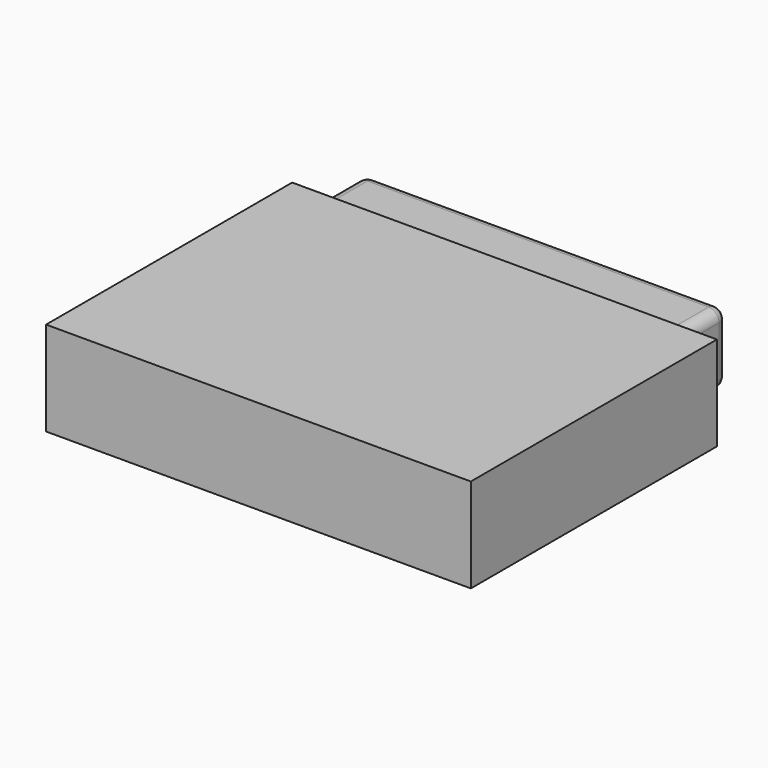
from build123d import *

# Parameters (mm, degrees)
F0_W         = 203
F0_H         = 147
F1_DEPTH     = 45
F2_R         = 7
F3_DEPTH     = 3
F4_R         = 9
F5_DEPTH     = 10
F6_W         = 173
F6_H         = 34
F7_DEPTH     = 25
F8_T1_DEPTH  = 163
F8_T3_DEPTH  = 24
F8_T5_DEPTH  = 20
F8_S9_W      = 5
F8_S9_H      = 5
F8_T10_DEPTH = 5
F8_S15_W     = 5
F8_S15_H     = 5
F8_T16_DEPTH = 5
F8_S21_W     = 5
F8_S21_H     = 5
F8_T22_DEPTH = 5
F8_S27_W     = 5
F8_S27_H     = 5
F8_T28_DEPTH = 5
F8_T34_DEPTH = 22.5
F8_S36_R     = 9
F8_T37_DEPTH = 13
F8_T42_DEPTH = 10
F8_S43_R     = 9
F8_T44_DEPTH = 8
F8_T48_DEPTH = 10
F8_S49_R     = 9
F8_T50_DEPTH = 8
F9_W         = 18
F9_H         = 30
F10_DEPTH    = 10


# Not quite as in the source:
# - a fillet or chamfer that OpenCascade refuses, or shapes differently, is made with other operations: its cross-section is extruded or revolved along the edge and cut away or added


with BuildPart() as f1:
    # F0 (on Top) → F1 (new body)
    with BuildSketch(Plane.XY):
        with Locations((0, 73.5)):
            Rectangle(F0_W, F0_H)
    extrude(amount=F1_DEPTH)

    # F2 (on face) → F3 (join)
    with BuildSketch(Plane(origin=(0, 0, 0), x_dir=(1, 0, 0), z_dir=(0, 0, -1))):
        with Locations((-88.5, -14)):
            Circle(F2_R)
        with Locations((-88.5, -117)):
            Circle(F2_R)
        with Locations((88.5, -14)):
            Circle(F2_R)
        with Locations((88.5, -117)):
            Circle(F2_R)
    extrude(amount=F3_DEPTH)

    # F4 (on face) → F5 (join)
    with BuildSketch(Plane(origin=(0, 147, 0), x_dir=(-1, 0, 0), z_dir=(0, 1, 0))):
        with Locations((91, 8)):
            Circle(F4_R)
    extrude(amount=F5_DEPTH)

    # F6 (on face) → F7 (join)
    with BuildSketch(Plane(origin=(0, 147, 0), x_dir=(-1, 0, 0), z_dir=(0, 1, 0))):
        with Locations((0, 27)):
            Rectangle(F6_W, F6_H)
    extrude(amount=F7_DEPTH)

    # F8: fillet of radius 5 on 8 edges, made by hand

    # F8_s2 → F8_t1 (cut)
    with BuildSketch(Plane.YZ.offset(-81.5)):
        with BuildLine():
            ThreePointArc((172, 39), (170.5355339059, 42.5355339059), (167, 44))
            Line((167, 44), (172, 44))
            Line((172, 44), (172, 39))
        make_face()
        with BuildLine():
            ThreePointArc((167, 10), (170.5355339059, 11.4644660941), (172, 15))
            Line((172, 15), (172, 10))
            Line((172, 10), (167, 10))
        make_face()
    extrude(amount=F8_T1_DEPTH, mode=Mode.SUBTRACT)

    # F8_s4 → F8_t3 (cut)
    with BuildSketch(Plane.XY.offset(15)):
        with BuildLine():
            ThreePointArc((81.5, 172), (85.0355339059, 170.5355339059), (86.5, 167))
            Line((86.5, 167), (86.5, 172))
            Line((86.5, 172), (81.5, 172))
        make_face()
        with BuildLine():
            ThreePointArc((-81.5, 172), (-85.0355339059, 170.5355339059), (-86.5, 167))
            Line((-86.5, 167), (-86.5, 172))
            Line((-86.5, 172), (-81.5, 172))
        make_face()
    extrude(amount=F8_T3_DEPTH, mode=Mode.SUBTRACT)

    # F8_s6 → F8_t5 (cut)
    with BuildSketch(Plane.XZ.offset(-167)):
        with BuildLine():
            ThreePointArc((86.5, 39), (85.0355339059, 42.5355339059), (81.5, 44))
            Line((81.5, 44), (86.5, 44))
            Line((86.5, 44), (86.5, 39))
        make_face()
        with BuildLine():
            ThreePointArc((81.5, 10), (85.0355339059, 11.4644660941), (86.5, 15))
            Line((86.5, 15), (86.5, 10))
            Line((86.5, 10), (81.5, 10))
        make_face()
        with BuildLine():
            ThreePointArc((-81.5, 44), (-85.0355339059, 42.5355339059), (-86.5, 39))
            Line((-86.5, 39), (-86.5, 44))
            Line((-86.5, 44), (-81.5, 44))
        make_face()
    extrude(amount=F8_T5_DEPTH, mode=Mode.SUBTRACT)


with BuildPart() as f8_tool8:
    # F8_s9 → F8_t10 (new body)
    with BuildSketch(Plane.XZ.offset(-167)):
        with Locations((-84, 41.5)):
            Rectangle(F8_S9_W, F8_S9_H)
    extrude(amount=-F8_T10_DEPTH)

    # F8_s11 → F8_t12 (revolve, cut)
    with BuildSketch(Plane(origin=(-81.5, 167, 39), x_dir=(0.7071067812, 0, -0.7071067812), z_dir=(0.7071067812, 0, 0.7071067812))):
        with BuildLine():
            ThreePointArc((0, -5), (5, 0), (0, 5))
            Line((0, 5), (0, -5))
        make_face()
    revolve(axis=Axis((-81.5, 167, 39), (0, 1, 0)), mode=Mode.SUBTRACT)


with BuildPart() as f1_1:
    add(f1.part)

    # F8_t7: cut F8_tool8
    add(f8_tool8.part, mode=Mode.SUBTRACT)


with BuildPart() as f8_tool14:
    # F8_s15 → F8_t16 (new body)
    with BuildSketch(Plane.XZ.offset(-167)):
        with Locations((84, 41.5)):
            Rectangle(F8_S15_W, F8_S15_H)
    extrude(amount=-F8_T16_DEPTH)

    # F8_s17 → F8_t18 (revolve, cut)
    with BuildSketch(Plane(origin=(81.5, 167, 39), x_dir=(-0.7071067812, 0, -0.7071067812), z_dir=(0.7071067812, 0, -0.7071067812))):
        with BuildLine():
            ThreePointArc((0, -5), (5, 0), (0, 5))
            Line((0, 5), (0, -5))
        make_face()
    revolve(axis=Axis((81.5, 167, 39), (0, 1, 0)), mode=Mode.SUBTRACT)


with BuildPart() as f1_2:
    add(f1_1.part)

    # F8_t13: cut F8_tool14
    add(f8_tool14.part, mode=Mode.SUBTRACT)


with BuildPart() as f8_tool20:
    # F8_s21 → F8_t22 (new body)
    with BuildSketch(Plane.XY.offset(15)):
        with Locations((84, 169.5)):
            Rectangle(F8_S21_W, F8_S21_H)
    extrude(amount=-F8_T22_DEPTH)

    # F8_s23 → F8_t24 (revolve, cut)
    with BuildSketch(Plane(origin=(81.5, 167, 15), x_dir=(-0.7071067812, -0.7071067812, 0), z_dir=(0.7071067812, -0.7071067812, 0))):
        with BuildLine():
            ThreePointArc((0, -5), (5, 0), (0, 5))
            Line((0, 5), (0, -5))
        make_face()
    revolve(axis=Axis((81.5, 167, 15), (0, 0, -1)), mode=Mode.SUBTRACT)


with BuildPart() as f1_3:
    add(f1_2.part)

    # F8_t19: cut F8_tool20
    add(f8_tool20.part, mode=Mode.SUBTRACT)


with BuildPart() as f8_tool26:
    # F8_s27 → F8_t28 (new body)
    with BuildSketch(Plane.XY.offset(15)):
        with Locations((-84, 169.5)):
            Rectangle(F8_S27_W, F8_S27_H)
    extrude(amount=-F8_T28_DEPTH)

    # F8_s29 → F8_t30 (revolve, cut)
    with BuildSketch(Plane(origin=(-81.5, 167, 15), x_dir=(0.7071067812, -0.7071067812, 0), z_dir=(0.7071067812, 0.7071067812, 0))):
        with BuildLine():
            ThreePointArc((0, -5), (5, 0), (0, 5))
            Line((0, 5), (0, -5))
        make_face()
    revolve(axis=Axis((-81.5, 167, 15), (0, 0, -1)), mode=Mode.SUBTRACT)


with BuildPart() as f1_4:
    add(f1_3.part)

    # F8_t25: cut F8_tool26
    add(f8_tool26.part, mode=Mode.SUBTRACT)


with BuildPart() as f8_tool32:
    # F8_s33 → F8_t34 (new body)
    with BuildSketch(Plane.XZ.offset(-144.5)):
        with BuildLine():
            ThreePointArc((-81.5, 10), (-85.0355339059, 11.4644660941), (-86.5, 15))
            Line((-86.5, 15), (-86.5, 10))
            Line((-86.5, 10), (-81.5, 10))
        make_face()
    extrude(amount=-F8_T34_DEPTH)

    split(bisect_by=Plane.XZ.offset(-147), keep=Keep.BOTTOM)

    # F8_s36 → F8_t37 (cut, symmetric)
    with BuildSketch(Plane.XZ.offset(-155.8)):
        with Locations((-91, 8)):
            Circle(F8_S36_R)
    extrude(amount=F8_T37_DEPTH, both=True, mode=Mode.SUBTRACT)

    split(bisect_by=Plane.XZ.offset(-157), keep=Keep.TOP)


with BuildPart() as f1_5:
    add(f1_4.part)

    # F8_t31: cut F8_tool32
    add(f8_tool32.part, mode=Mode.SUBTRACT)


with BuildPart() as f8_tool40:
    # F8_s41 → F8_t42 (new body)
    with BuildSketch(Plane.XZ.offset(-157)):
        with BuildLine():
            ThreePointArc((-81.5, 10), (-85.0355339059, 11.4644660941), (-86.5, 15))
            Line((-86.5, 15), (-86.5, 10))
            Line((-86.5, 10), (-81.5, 10))
        make_face()
    extrude(amount=-F8_T42_DEPTH)

    # F8_s43 → F8_t44 (cut, symmetric)
    with BuildSketch(Plane.XZ.offset(-162)):
        with Locations((-91, 8)):
            Circle(F8_S43_R)
    extrude(amount=F8_T44_DEPTH, both=True, mode=Mode.SUBTRACT)


with BuildPart() as f1_6:
    add(f1_5.part)

    # F8_t39: cut F8_tool40
    add(f8_tool40.part, mode=Mode.SUBTRACT)


with BuildPart() as f8_tool46:
    # F8_s47 → F8_t48 (new body)
    with BuildSketch(Plane.XZ.offset(-157)):
        with BuildLine():
            ThreePointArc((-81.5, 10), (-85.0355339059, 11.4644660941), (-86.5, 15))
            Line((-86.5, 15), (-86.5, 10))
            Line((-86.5, 10), (-81.5, 10))
        make_face()
    extrude(amount=-F8_T48_DEPTH)

    # F8_s49 → F8_t50 (intersect, symmetric)
    with BuildSketch(Plane.XZ.offset(-162)):
        with Locations((-91, 8)):
            Circle(F8_S49_R)
    extrude(amount=F8_T50_DEPTH, both=True, mode=Mode.INTERSECT)


with BuildPart() as f1_7:
    add(f1_6.part)

    # F8_t45: cut F8_tool46
    add(f8_tool46.part, mode=Mode.SUBTRACT)

    # F9 (on face) → F10 (join, through all)
    with BuildSketch(Plane(origin=(0, 157, 0), x_dir=(-1, 0, 0), z_dir=(0, 1, 0))):
        with Locations((91, 23)):
            Rectangle(F9_W, F9_H)
    extrude(amount=-F10_DEPTH)


solid = f1_7.part
